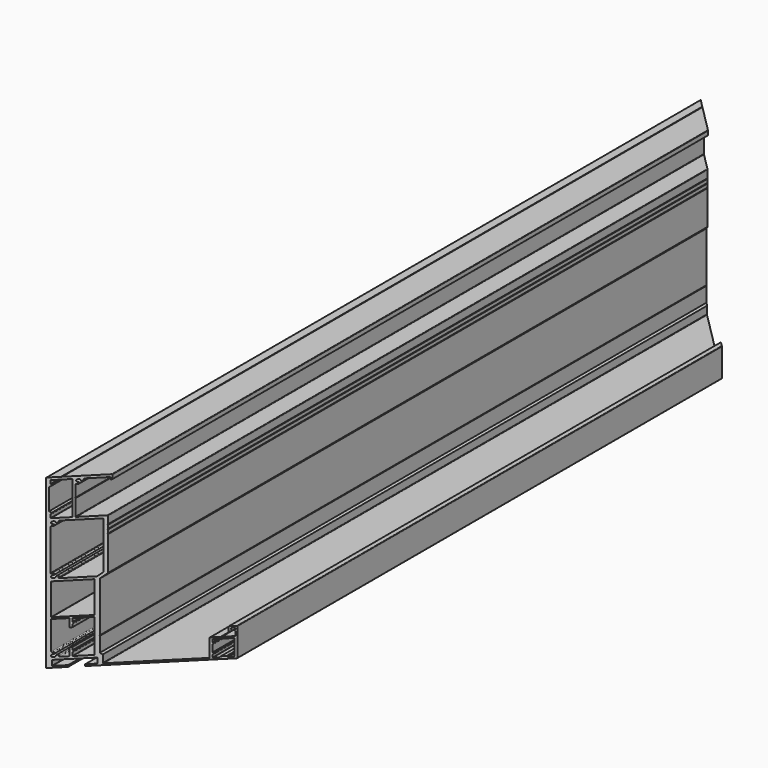
from build123d import *

# Parameters (mm, degrees)
F1_DEPTH = 500
F3_DEPTH = 205.001


# Not quite as in the source:
# - ends of sketch curves that miss each other by under 0.0002 mm in the source are joined


with BuildPart() as f1:
    # F0 (on Front) → F1 (new body, symmetric)
    with BuildSketch(Plane.XZ):
        with BuildLine():
            Line((124.375184, 29.377061), (124.9560899959, 29.377061))
            ThreePointArc((124.9560899959, 29.377061), (124.968792, 29.37698), (124.9814940041, 29.3770606737))
            Line((124.9814940041, 29.3770606737), (125.505952, 29.377061))
            ThreePointArc((125.505952, 29.377061), (125.5111512264, 29.4913383789), (125.5781343153, 29.5840725896))
            ThreePointArc((125.5781343153, 29.5840725896), (125.9612588099, 30.2544614615), (125.7526842073, 30.9979011642))
            ThreePointArc((125.7526842073, 30.9979011642), (127, 33.6), (128.2473160951, 30.9979009236))
            ThreePointArc((128.2473160951, 30.9979009236), (128.0387411901, 30.2544614615), (128.4218653386, 29.5840721393))
            ThreePointArc((128.4218653386, 29.5840721393), (128.479406155, 29.513882617), (128.5, 29.425489))
            Line((128.5, 29.425489), (128.5, 24.5))
            ThreePointArc((128.5, 24.5), (128.3535533906, 24.1464466094), (128, 24))
            Line((128, 24), (119.225184, 24))
            Line((119.225184, 24), (118.875184, 23.65))
            Line((118.875184, 23.65), (118.525184, 24))
            Line((118.525184, 24), (111.5, 24))
            ThreePointArc((111.5, 24), (111.1464466094, 23.8535533906), (111, 23.5))
            Line((111, 23.5), (111, 2.5))
            ThreePointArc((111, 2.5), (110.8535533906, 2.1464466094), (110.5, 2))
            Line((110.5, 2), (38.984614, 2))
            ThreePointArc((38.984614, 2), (38.6310606094, 2.1464466094), (38.484614, 2.5))
            Line((38.484614, 2.5), (38.484614, 11.290435))
            ThreePointArc((38.484614, 11.290435), (38.4465537663, 11.4817767162), (38.3381673906, 11.6439883906))
            Line((38.3381673906, 11.6439883906), (36.648572, 13.333584))
            ThreePointArc((36.648572, 13.333584), (36.540185369, 13.4957959572), (36.502125, 13.687138))
            Line((36.502125, 13.687138), (36.502125, 31.647489))
            Line((36.502125, 31.647489), (36.152125, 31.997489))
            Line((36.152125, 31.997489), (36.502125, 32.347489))
            Line((36.502125, 32.347489), (36.502125, 93.210624))
            ThreePointArc((36.502125, 93.210624), (36.5401852337, 93.4019657162), (36.6485716094, 93.5641773906))
            Line((36.6485716094, 93.5641773906), (41.856953, 98.772559))
            ThreePointArc((41.856953, 98.772559), (41.9653397663, 98.9347702838), (42.0034, 99.126112))
            Line((42.0034, 99.126112), (42.0034, 140.65))
            Line((42.0034, 140.65), (41.6534, 141))
            Line((41.6534, 141), (42.0034, 141.35))
            Line((42.0034, 141.35), (42.0034, 145.65))
            Line((42.0034, 145.65), (41.6534, 146))
            Line((41.6534, 146), (42.0034, 146.35))
            Line((42.0034, 146.35), (42.0034, 150.65))
            Line((42.0034, 150.65), (41.6534, 151))
            Line((41.6534, 151), (42.0034, 151.35))
            Line((42.0034, 151.35), (42.0034, 160.5))
            ThreePointArc((42.0034, 160.5), (41.8569533906, 160.8535533906), (41.5034, 161))
            Line((41.5034, 161), (20.5, 161))
            ThreePointArc((20.5, 161), (20.1464466094, 161.1464466094), (20, 161.5))
            Line((20, 161.5), (20, 181.15))
            Line((20, 181.15), (19.65, 181.5))
            Line((19.65, 181.5), (20, 181.85))
            Line((20, 181.85), (20, 195.92334))
            ThreePointArc((20, 195.92334), (20.1464466094, 196.2768933906), (20.5, 196.42334))
            Line((20.5, 196.42334), (21.7882, 196.42334))
            ThreePointArc((21.7882, 196.42334), (22.7653211867, 197.3573315865), (21.8763609796, 198.3755927746))
            ThreePointArc((21.8763609796, 198.3755927746), (20.8418899384, 201.1457592182), (23.6229875458, 200.1410479605))
            ThreePointArc((23.6229875458, 200.1410479605), (24.6339421806, 199.2343237784), (25.57666, 200.2118))
            Line((25.57666, 200.2118), (25.57666, 201.5))
            ThreePointArc((25.57666, 201.5), (25.7231066094, 201.8535533906), (26.07666, 202))
            Line((26.07666, 202), (43.2, 202))
            ThreePointArc((43.2, 202), (43.5535533906, 201.8535533906), (43.7, 201.5))
            Line((43.7, 201.5), (43.7, 199.7))
            ThreePointArc((43.7, 199.7), (43.7585786438, 199.5585786438), (43.9, 199.5))
            Line((43.9, 199.5), (44.8, 199.5))
            ThreePointArc((44.8, 199.5), (44.9414213562, 199.5585786438), (45, 199.7))
            Line((45, 199.7), (45, 204.5))
            ThreePointArc((45, 204.5), (44.8535533906, 204.8535533906), (44.5, 205))
            Line((44.5, 205), (10.9, 205))
            Line((10.9, 205), (10.55, 204.65))
            Line((10.55, 204.65), (10.2, 205))
            Line((10.2, 205), (0.5, 205))
            ThreePointArc((0.5, 205), (0.1464466094, 204.8535533906), (0, 204.5))
            Line((0, 204.5), (0, 0.5))
            ThreePointArc((0, 0.5), (0.1464466094, 0.1464466094), (0.5, 0))
            Line((0.5, 0), (14.862233, 0))
            ThreePointArc((14.862233, 0), (15.0036543562, 0.0585786438), (15.062233, 0.2))
            Line((15.062233, 0.2), (15.062233, 1.8))
            ThreePointArc((15.062233, 1.8), (15.0036543562, 1.9414213562), (14.862233, 2))
            Line((14.862233, 2), (4.184648, 2))
            ThreePointArc((4.184648, 2), (4.0432266438, 2.0585786438), (3.984648, 2.2))
            Line((3.984648, 2.2), (3.984648, 8.3))
            ThreePointArc((3.984648, 8.3), (4.0432266438, 8.4414213562), (4.184648, 8.5))
            Line((4.184648, 8.5), (25.439573, 8.5))
            Line((25.439573, 8.5), (25.789573, 8.85))
            Line((25.789573, 8.85), (26.139573, 8.5))
            Line((26.139573, 8.5), (34.784648, 8.5))
            ThreePointArc((34.784648, 8.5), (34.9260693562, 8.4414213562), (34.984648, 8.3))
            Line((34.984648, 8.3), (34.984648, 2.2))
            ThreePointArc((34.984648, 2.2), (34.9260693562, 2.0585786438), (34.784648, 2))
            Line((34.784648, 2), (26.583975, 2))
            ThreePointArc((26.583975, 2), (26.4425536438, 1.9414213562), (26.383975, 1.8))
            Line((26.383975, 1.8), (26.383975, 0.2))
            ThreePointArc((26.383975, 0.2), (26.4425536438, 0.0585786438), (26.583975, 0))
            Line((26.583975, 0), (129.5, 0))
            ThreePointArc((129.5, 0), (129.8535533906, 0.1464466094), (130, 0.5))
            Line((130, 0.5), (130, 34.5))
            ThreePointArc((130, 34.5), (129.8535533906, 34.8535533906), (129.5, 35))
            Line((129.5, 35), (124.375184, 35))
            ThreePointArc((124.375184, 35), (124.0216306094, 34.8535533906), (123.875184, 34.5))
            Line((123.875184, 34.5), (123.875184, 29.877061))
            ThreePointArc((123.875184, 29.877061), (124.0216306094, 29.5235076094), (124.375184, 29.377061))
        make_face()
        with BuildLine():
            Line((32.939573, 52.297501), (32.939573, 51.997501))
            Line((32.939573, 51.997501), (32.939573, 11.997478))
            Line((32.939573, 11.997478), (32.939573, 11.697478))
            ThreePointArc((32.939573, 11.697478), (32.8809943562, 11.5560566438), (32.739573, 11.497478))
            Line((32.739573, 11.497478), (18.239573, 11.497478))
            ThreePointArc((18.239573, 11.497478), (18.0981516438, 11.5560566438), (18.039573, 11.697478))
            Line((18.039573, 11.697478), (18.039573, 15.609124))
            ThreePointArc((18.039573, 15.609124), (18.0547970935, 15.6856606865), (18.0981516438, 15.7505453562))
            Line((18.0981516438, 15.7505453562), (18.580995, 16.233388))
            ThreePointArc((18.580995, 16.233388), (18.6243490418, 16.2982726402), (18.639573, 16.374809))
            Line((18.639573, 16.374809), (18.639573, 17.209124))
            ThreePointArc((18.639573, 17.209124), (18.6243490418, 17.2856603598), (18.5809948562, 17.3505448562))
            Line((18.5809948562, 17.3505448562), (18.098152, 17.833388))
            ThreePointArc((18.098152, 17.833388), (18.0547970935, 17.8982723135), (18.039573, 17.974809))
            Line((18.039573, 17.974809), (18.039573, 21.297478))
            ThreePointArc((18.039573, 21.297478), (17.9809943562, 21.4388993562), (17.839573, 21.497478))
            Line((17.839573, 21.497478), (16.25286, 21.497478))
            ThreePointArc((16.25286, 21.497478), (16.1114386438, 21.4388993562), (16.05286, 21.297478))
            Line((16.05286, 21.297478), (16.05286, 11.997461))
            ThreePointArc((16.05286, 11.997461), (15.9064194009, 11.6439136199), (15.552877, 11.4974610003))
            Line((15.552877, 11.4974610003), (9.576694, 11.497255))
            ThreePointArc((9.576694, 11.497255), (8.8695652397, 11.7901361981), (8.57666, 12.497255))
            Line((8.57666, 12.497255), (8.57666, 12.7882))
            ThreePointArc((8.57666, 12.7882), (7.6339421806, 13.7656762216), (6.6229882742, 12.8589519801))
            ThreePointArc((6.6229882742, 12.8589519801), (3.8418899384, 11.8542407818), (4.8763610373, 14.6244065094))
            ThreePointArc((4.8763610373, 14.6244065094), (5.7653211867, 15.6426684135), (4.7882, 16.57666))
            Line((4.7882, 16.57666), (4.5, 16.57666))
            ThreePointArc((4.5, 16.57666), (3.7928932188, 16.8695532188), (3.5, 17.57666))
            Line((3.5, 17.57666), (3.5, 52.297501))
            ThreePointArc((3.5, 52.297501), (3.5585786438, 52.4389223562), (3.7, 52.497501))
            Line((3.7, 52.497501), (15.85286, 52.497501))
            ThreePointArc((15.85286, 52.497501), (15.9942813562, 52.4389223562), (16.05286, 52.297501))
            Line((16.05286, 52.297501), (16.05286, 42.697501))
            ThreePointArc((16.05286, 42.697501), (16.1114386438, 42.5560796438), (16.25286, 42.497501))
            Line((16.25286, 42.497501), (17.839573, 42.497501))
            ThreePointArc((17.839573, 42.497501), (17.9809943562, 42.5560796438), (18.039573, 42.697501))
            Line((18.039573, 42.697501), (18.039573, 46.02017))
            ThreePointArc((18.039573, 46.02017), (18.0547970935, 46.0967066865), (18.0981516438, 46.1615913562))
            Line((18.0981516438, 46.1615913562), (18.580995, 46.644434))
            ThreePointArc((18.580995, 46.644434), (18.6243490418, 46.7093186402), (18.639573, 46.785855))
            Line((18.639573, 46.785855), (18.639573, 47.62017))
            ThreePointArc((18.639573, 47.62017), (18.6243490418, 47.6967063598), (18.5809948562, 47.7615908562))
            Line((18.5809948562, 47.7615908562), (18.098152, 48.244434))
            ThreePointArc((18.098152, 48.244434), (18.0547970935, 48.3093183135), (18.039573, 48.385855))
            Line((18.039573, 48.385855), (18.039573, 52.297501))
            ThreePointArc((18.039573, 52.297501), (18.0981516438, 52.4389223562), (18.239573, 52.497501))
            Line((18.239573, 52.497501), (32.739573, 52.497501))
            ThreePointArc((32.739573, 52.497501), (32.8809943562, 52.4389223562), (32.939573, 52.297501))
        make_face(mode=Mode.SUBTRACT)
        with BuildLine():
            ThreePointArc((3.7, 54.469528), (3.5585786438, 54.5281066438), (3.5, 54.669528))
            Line((3.5, 54.669528), (3.5, 92.8))
            ThreePointArc((3.5, 92.8), (3.5585786438, 92.9414213562), (3.7, 93))
            Line((3.7, 93), (32.739573, 93))
            ThreePointArc((32.739573, 93), (32.8809943562, 92.9414213562), (32.939573, 92.8))
            Line((32.939573, 92.8), (32.939573, 54.669528))
            ThreePointArc((32.939573, 54.669528), (32.8809943562, 54.5281066438), (32.739573, 54.469528))
            Line((32.739573, 54.469528), (3.7, 54.469528))
        make_face(mode=Mode.SUBTRACT)
        with BuildLine():
            Line((123.441776, 2.058579), (122.558934, 2.941421))
            ThreePointArc((122.558934, 2.941421), (122.4940490131, 2.9847757712), (122.417512, 3))
            Line((122.417512, 3), (118.583198, 3))
            ThreePointArc((118.583198, 3), (118.5066609869, 2.9847757712), (118.4417761438, 2.9414208562))
            Line((118.4417761438, 2.9414208562), (117.558934, 2.058579))
            ThreePointArc((117.558934, 2.058579), (117.4940490131, 2.0152242288), (117.417512, 2))
            Line((117.417512, 2), (113.20071, 2))
            ThreePointArc((113.20071, 2), (113.0592886438, 2.0585786438), (113.00071, 2.2))
            Line((113.00071, 2.2), (113.00071, 5.217867))
            ThreePointArc((113.00071, 5.217867), (113.0159342288, 5.2944040131), (113.0592891438, 5.3592888562))
            Line((113.0592891438, 5.3592888562), (113.641421, 5.941421))
            ThreePointArc((113.641421, 5.941421), (113.6847757712, 6.0063059869), (113.7, 6.082843))
            Line((113.7, 6.082843), (113.7, 6.917157))
            ThreePointArc((113.7, 6.917157), (113.6847757712, 6.9936940131), (113.6414208562, 7.0585788562))
            Line((113.6414208562, 7.0585788562), (113.059289, 7.640711))
            ThreePointArc((113.059289, 7.640711), (113.0159342288, 7.7055959869), (113.00071, 7.782133))
            Line((113.00071, 7.782133), (113.00071, 16.217867))
            ThreePointArc((113.00071, 16.217867), (113.0159342288, 16.2944040131), (113.0592891438, 16.3592888562))
            Line((113.0592891438, 16.3592888562), (113.641421, 16.941421))
            ThreePointArc((113.641421, 16.941421), (113.6847757712, 17.0063059869), (113.7, 17.082843))
            Line((113.7, 17.082843), (113.7, 17.917157))
            ThreePointArc((113.7, 17.917157), (113.6847757712, 17.9936940131), (113.6414208562, 18.0585788562))
            Line((113.6414208562, 18.0585788562), (113.059289, 18.640711))
            ThreePointArc((113.059289, 18.640711), (113.0159342288, 18.7055959869), (113.00071, 18.782133))
            Line((113.00071, 18.782133), (113.00071, 21.8))
            ThreePointArc((113.00071, 21.8), (113.0592886438, 21.9414213562), (113.20071, 22))
            Line((113.20071, 22), (127.8, 22))
            ThreePointArc((127.8, 22), (127.9414213562, 21.9414213562), (128, 21.8))
            Line((128, 21.8), (128, 2.2))
            ThreePointArc((128, 2.2), (127.9414213562, 2.0585786438), (127.8, 2))
            Line((127.8, 2), (123.583198, 2))
            ThreePointArc((123.583198, 2), (123.5066609869, 2.0152242288), (123.441776, 2.058579))
        make_face(mode=Mode.SUBTRACT)
        with BuildLine():
            ThreePointArc((9.07666, 96), (8.7231066094, 96.1464466094), (8.57666, 96.5))
            Line((8.57666, 96.5), (8.57666, 97.7882))
            ThreePointArc((8.57666, 97.7882), (7.6339421806, 98.7656762216), (6.6229882742, 97.8589519801))
            ThreePointArc((6.6229882742, 97.8589519801), (3.8418899384, 96.8542407818), (4.8763610373, 99.6244065094))
            ThreePointArc((4.8763610373, 99.6244065094), (5.7653211867, 100.6426684135), (4.7882, 101.57666))
            Line((4.7882, 101.57666), (3.5, 101.57666))
            ThreePointArc((3.5, 101.57666), (3.1464466094, 101.7231066094), (3, 102.07666))
            Line((3, 102.07666), (3, 151.92334))
            ThreePointArc((3, 151.92334), (3.1464466094, 152.2768933906), (3.5, 152.42334))
            Line((3.5, 152.42334), (4.7882, 152.42334))
            ThreePointArc((4.7882, 152.42334), (5.7653211867, 153.3573315865), (4.8763609796, 154.3755927746))
            ThreePointArc((4.8763609796, 154.3755927746), (3.8418899384, 157.1457592182), (6.6229875458, 156.1410479605))
            ThreePointArc((6.6229875458, 156.1410479605), (7.6339421806, 155.2343237784), (8.57666, 156.2118))
            Line((8.57666, 156.2118), (8.57666, 157.5))
            ThreePointArc((8.57666, 157.5), (8.7231066094, 157.8535533906), (9.07666, 158))
            Line((9.07666, 158), (38.5, 158))
            ThreePointArc((38.5, 158), (38.8535533906, 157.8535533906), (39, 157.5))
            Line((39, 157.5), (39, 100.42726))
            ThreePointArc((39, 100.42726), (38.9619397663, 100.2359182838), (38.8535533906, 100.0737066094))
            Line((38.8535533906, 100.0737066094), (34.926293, 96.146447))
            ThreePointArc((34.926293, 96.146447), (34.7640817162, 96.0380602337), (34.57274, 96))
            Line((34.57274, 96), (9.07666, 96))
        make_face(mode=Mode.SUBTRACT)
        with BuildLine():
            Line((17.8, 161), (3.3, 161))
            ThreePointArc((3.3, 161), (3.1585786438, 161.0585786438), (3.1, 161.2))
            Line((3.1, 161.2), (3.1, 165.111646))
            ThreePointArc((3.1, 165.111646), (3.1152242288, 165.1881830131), (3.1585791438, 165.2530678562))
            Line((3.1585791438, 165.2530678562), (3.641421, 165.73591))
            ThreePointArc((3.641421, 165.73591), (3.6847757712, 165.8007949869), (3.7, 165.877332))
            Line((3.7, 165.877332), (3.7, 166.711646))
            ThreePointArc((3.7, 166.711646), (3.6847757712, 166.7881830131), (3.6414208562, 166.8530678562))
            Line((3.6414208562, 166.8530678562), (2.146447, 168.348042))
            ThreePointArc((2.146447, 168.348042), (2.038060369, 168.5102539572), (2, 168.701596))
            Line((2, 168.701596), (2, 194.298404))
            ThreePointArc((2, 194.298404), (2.038060369, 194.4897460428), (2.1464471094, 194.6519578906))
            Line((2.1464471094, 194.6519578906), (3.641421, 196.146932))
            ThreePointArc((3.641421, 196.146932), (3.6847757712, 196.2118169869), (3.7, 196.288354))
            Line((3.7, 196.288354), (3.7, 197.122668))
            ThreePointArc((3.7, 197.122668), (3.6847757712, 197.1992050131), (3.6414208562, 197.2640898562))
            Line((3.6414208562, 197.2640898562), (3.158579, 197.746932))
            ThreePointArc((3.158579, 197.746932), (3.1152242288, 197.8118169869), (3.1, 197.888354))
            Line((3.1, 197.888354), (3.1, 201.8))
            ThreePointArc((3.1, 201.8), (3.1585786438, 201.9414213562), (3.3, 202))
            Line((3.3, 202), (17.8, 202))
            ThreePointArc((17.8, 202), (17.9414213562, 201.9414213562), (18, 201.8))
            Line((18, 201.8), (18, 161.2))
            ThreePointArc((18, 161.2), (17.9414213562, 161.0585786438), (17.8, 161))
        make_face(mode=Mode.SUBTRACT)
    extrude(amount=F1_DEPTH, both=True)

    # F2 (on face) → F3 (cut, through all)
    with BuildSketch(Plane(origin=(0, 0, 0), x_dir=(1, 0, 0), z_dir=(0, 0, -1))):
        Polygon((130, 500), (0, 500), (130, 370), align=None)
        Polygon((0, -500), (130, -500), (130, -370), align=None)
    extrude(amount=-F3_DEPTH, mode=Mode.SUBTRACT)


solid = f1.part
